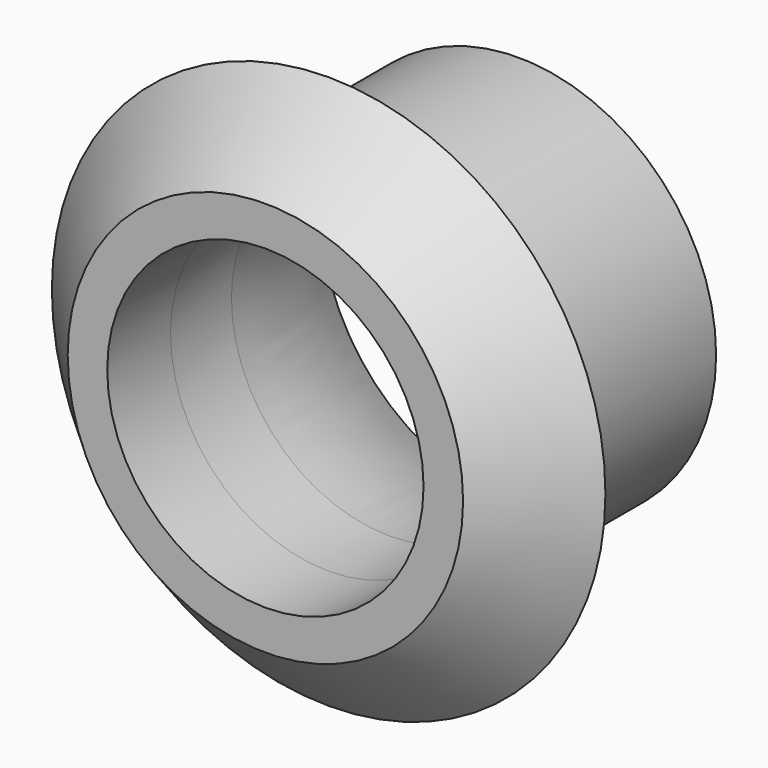
from build123d import *

# Parameters (mm, degrees)
F0_R     = 17.5
F0_R_2   = 12.5
F0_R_3   = 10
F1_DEPTH = 5
F2_DEPTH = 15
F4_SIZE  = 4.99999


# Not quite as in the source:
# - a fillet or chamfer that OpenCascade refuses, or shapes differently, is made with other operations: its cross-section is extruded or revolved along the edge and cut away or added
# - a fillet or chamfer is up to 0.001 mm smaller than in the source, because OpenCascade refuses the exact size


with BuildPart() as f1:
    # F0 (on Front) → F1 (new body)
    with BuildSketch(Plane.XZ):
        Circle(F0_R)
        Circle(F0_R_2, mode=Mode.SUBTRACT)
        Circle(F0_R_2)
        Circle(F0_R_3, mode=Mode.SUBTRACT)
    extrude(amount=F1_DEPTH)

    # F0 (on Front) → F2 (join)
    with BuildSketch(Plane.XZ):
        Circle(F0_R_2)
        Circle(F0_R_3, mode=Mode.SUBTRACT)
    extrude(amount=-F2_DEPTH)

    # F3: fillet of radius 22 on 1 edges, made by hand

    # F3_s1 → F3_t2 (revolve, cut)
    with BuildSketch(Plane.XY):
        with BuildLine():
            ThreePointArc((10, 4.8142256063), (10.6341393808, 10.0582698471), (12.5, 15))
            Line((12.5, 15), (10, 15))
            Line((10, 15), (10, 4.8142256063))
        make_face()
    revolve(axis=Axis((0, 15, 0), (0, -1, 0)), mode=Mode.SUBTRACT)

    # F4 (size 5 in the source; OpenCascade refuses exactly that, so slightly less here)
    f4_edges = [f1.edges().sort_by_distance(p)[0] for p in [
        (-17.5, -5, 0),
    ]]
    chamfer(f4_edges, length=F4_SIZE)


solid = f1.part
